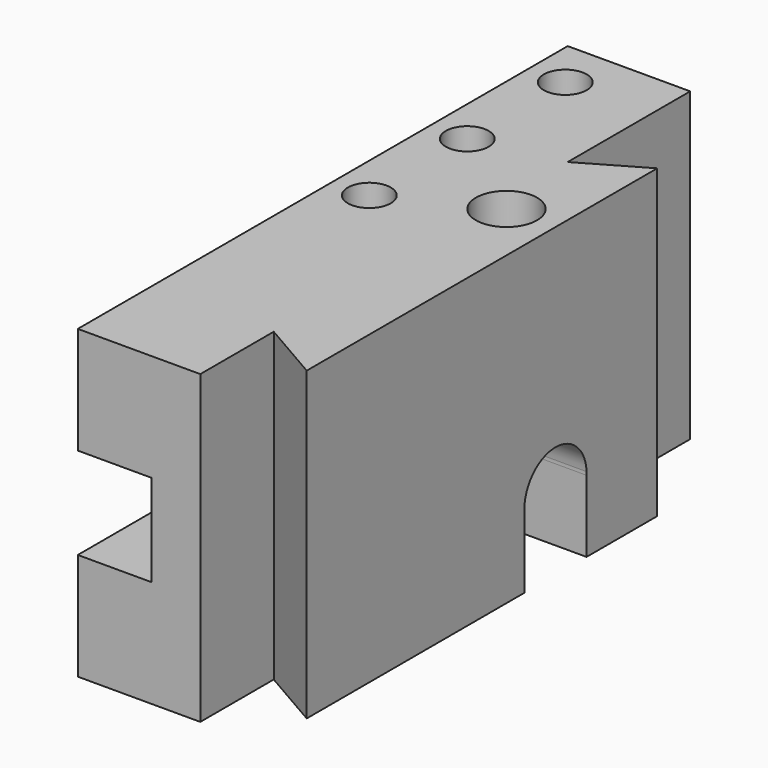
from build123d import *

# Parameters (mm, degrees)
F1_DEPTH = 31.75
F2_W     = 15.24
F2_H     = 9.525
F3_DEPTH = 63.501
F4_R     = 2.2225
F5_DEPTH = 11.1125
F6_R     = 3.175
F7_DEPTH = 25.4
F9_DEPTH = 10.16


# Not quite as in the source:
# - a feature names something its author has since deleted; it is built from what else it names


with BuildPart() as f1:
    # F0 (on Top) → F1 (new body)
    with BuildSketch(Plane.XY):
        Polygon((3.175, 31.75), (-9.525, 31.75), (-9.525, -31.75), (3.175, -31.75), (3.175, -22.225), (3.175, 15.875), align=None)
        Polygon((9.525, 19.5411742094), (3.175, 15.875), (3.175, -22.225), (9.525, -25.8911742094), align=None)
    extrude(amount=F1_DEPTH)

    # F2 (on face) → F3 (cut, through all)
    with BuildSketch(Plane.XZ.offset(31.75)):
        with Locations((-9.525, 15.875)):
            Rectangle(F2_W, F2_H)
    extrude(amount=-F3_DEPTH, mode=Mode.SUBTRACT)

    # F4 (on face) → F5 (cut, through all)
    with BuildSketch(Plane.XY.offset(31.75)):
        with Locations((-5.715, 1.27)):
            Circle(F4_R)
        with Locations((-5.715, 13.97)):
            Circle(F4_R)
        with Locations((-5.715, 26.67)):
            Circle(F4_R)
    extrude(amount=-F5_DEPTH, mode=Mode.SUBTRACT)

    # F6 (on face) → F7 (cut)
    with BuildSketch(Plane.XY.offset(31.75)):
        with Locations((4.445, 6.35)):
            Circle(F6_R)
    extrude(amount=-F7_DEPTH, mode=Mode.SUBTRACT)

    # F8 (on face) → F9 (cut)
    with BuildSketch(Plane.YZ.offset(9.525)):
        with BuildLine():
            Line((10.3787716824, 7.7874478821), (10.3787716824, 7.4525521179))
            ThreePointArc((10.3787716824, 7.4525521179), (10.38225, 7.62), (10.3787716824, 7.7874478821))
        make_face()
        with BuildLine():
            Line((10.3787716824, 0), (10.3787716824, 7.4525521179))
            Line((10.3787716824, 7.4525521179), (10.3787716824, 7.7874478821))
            ThreePointArc((10.3787716824, 7.7874478821), (6.2662579975, 11.6513803268), (2.31775, 7.62))
            Line((2.31775, 7.62), (2.31775, 0))
            Line((2.31775, 0), (10.3787716824, 0))
        make_face()
    extrude(amount=-F9_DEPTH, mode=Mode.SUBTRACT)


solid = f1.part
